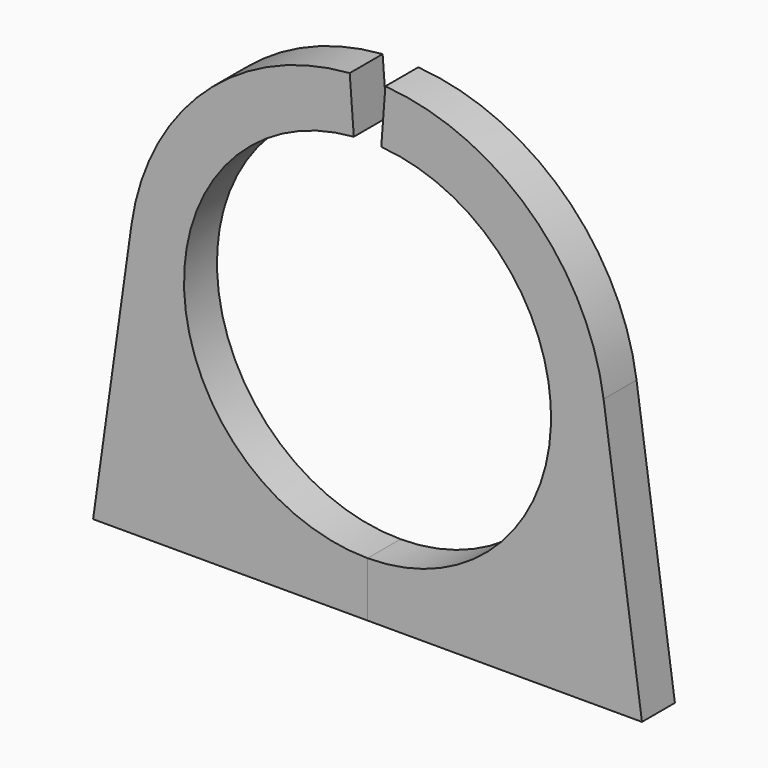
from build123d import *
from build123d import SkipClean  # not in build123d's __all__

# Parameters (mm, degrees)
F1_DEPTH = 6


with BuildPart() as f1:
    # F0 (on Front) → F1 (new body)
    with BuildSketch(Plane.XZ):
        with BuildLine():
            ThreePointArc((-2.5981308411, 69.4027374984), (-23.7554424043, 60.1122052703), (-34.4088510941, 39.607310612))
            Line((-34.4088510941, 39.607310612), (-40, 0))
            Line((-40, 0), (0, 0))
            Line((0, 0), (0, 8))
            ThreePointArc((0, 8), (-26.7312756631, 33.7492995345), (-2, 61.4251288657))
            Line((-2, 61.4251288657), (-2.5981308411, 69.4027374984))
        make_face()
    extrude(amount=F1_DEPTH)

    # F2: F1 across plane


with BuildPart() as f1_1:
    add(f1.part, clean=False)
    with SkipClean():  # cleaning this boolean's faces spoils the solid; the shape is the same uncleaned
        add(f1.part.mirror(Plane.YZ), clean=False)


solid = f1_1.part
